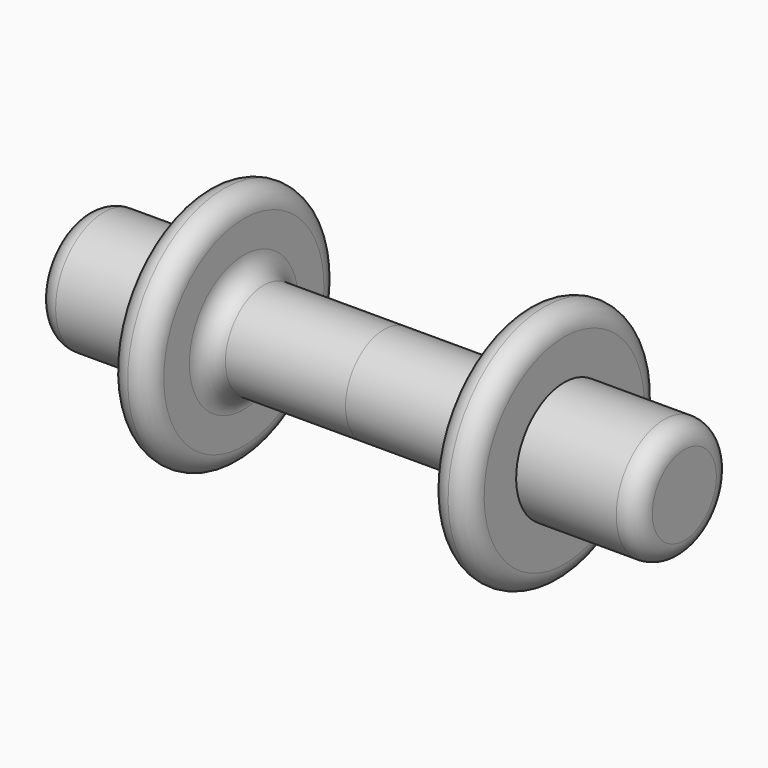
from build123d import *

# Parameters (mm, degrees)
F3_R = 4.99999


# Not quite as in the source:
# - a fillet or chamfer is up to 0.001 mm smaller than in the source, because OpenCascade refuses the exact size


with BuildPart() as f1:
    # F0 (on Front) → F1 (revolve)
    with BuildSketch(Plane.XZ):
        with BuildLine():
            Line((30, 12), (0, 12))
            Line((0, 12), (0, 0))
            Line((0, 0), (75, 0))
            Line((75, 0), (75, 15))
            Line((75, 15), (45, 15))
            Line((45, 15), (45, 30))
            Line((45, 30), (35, 30))
            Line((35, 30), (35, 17))
            ThreePointArc((35, 17), (33.5355339059, 13.4644660941), (30, 12))
        make_face()
    revolve(axis=Axis((37.5, 0, 0), (-1, 0, 0)))

    # F2: F1 across face


with BuildPart() as f1_1:
    add(f1.part)
    add(f1.part.mirror(Plane(origin=(0, 0, 0), x_dir=(0, -1, 0), z_dir=(-1, 0, 0))))

    # F3 (radius 5 in the source; OpenCascade refuses exactly that, so slightly less here)
    f3_edges = [f1_1.edges().sort_by_distance(p)[0] for p in [
        (75, 0, -15),
        (-75, 0, -15),
        (-35, 0, -30),
        (-45, 0, -30),
        (45, 0, -30),
        (35, 0, -30),
        (30, 0, -12),
        (0, 0, 12),
        (-30, 0, -12),
    ]]
    fillet(f3_edges, radius=F3_R)


solid = f1_1.part
